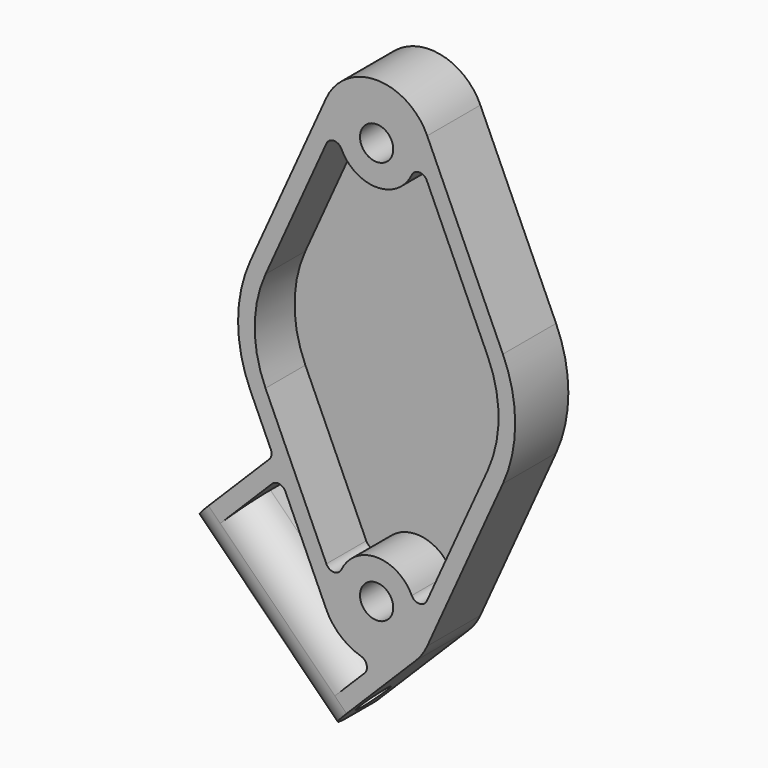
from build123d import *

# Parameters (mm, degrees)
F0_R     = 2
F1_DEPTH = 8
F2_DEPTH = 2
F3_R     = 1
F5_D     = 4
F6_R     = 3.99999


# Not quite as in the source:
# - a fillet or chamfer is up to 0.001 mm smaller than in the source, because OpenCascade refuses the exact size


with BuildPart() as f1:
    # F0 (on Front) → F1 (new body)
    with BuildSketch(Plane.XZ):
        with BuildLine():
            Line((15.1970139668, 6.8636525628), (6.0880650012, 27.0320429916))
            ThreePointArc((6.0880650012, 27.0320429916), (0, 30.9626), (-6.0880650012, 27.0320429916))
            Line((-6.0880650012, 27.0320429916), (-15.1970139668, 6.8636525628))
            ThreePointArc((-15.1970139668, 6.8636525628), (-16.6751, 0), (-15.1970139668, -6.8636525628))
            Line((-15.1970139668, -6.8636525628), (-12.4500889322, -12.9456996558))
            Line((-12.4500889322, -12.9456996558), (-11.570090993, -14.8941288413))
            Line((-11.570090993, -14.8941288413), (-6.0880650012, -27.0320429916))
            ThreePointArc((-6.0880650012, -27.0320429916), (-3.6489564687, -29.8779507977), (-0.0611180905, -30.9623204051))
            ThreePointArc((-0.0611180905, -30.9623204051), (2.5281419438, -30.4657300374), (4.7236147197, -29.0060147197))
            ThreePointArc((4.7236147197, -29.0060147197), (5.4952020611, -28.0807978659), (6.0880650012, -27.0320429916))
            Line((6.0880650012, -27.0320429916), (15.1970139668, -6.8636525628))
            ThreePointArc((15.1970139668, -6.8636525628), (16.6751, 0), (15.1970139668, 6.8636525628))
        make_face()
        with Locations((0, -24.2824)):
            Circle(F0_R, mode=Mode.SUBTRACT)
        with BuildLine():
            Line((-13.3742945868, 6.0404308054), (-6.0462846285, 22.2655920687))
            ThreePointArc((-6.0462846285, 22.2655920687), (-5.1436901116, 22.8539427752), (-4.2309206889, 22.2815046593))
            ThreePointArc((-4.2309206889, 22.2815046593), (0, 19.6022), (4.2309206889, 22.2815046593))
            ThreePointArc((4.2309206889, 22.2815046593), (5.1436901116, 22.8539427752), (6.0462846285, 22.2655920687))
            Line((6.0462846285, 22.2655920687), (13.3742945868, 6.0404308054))
            ThreePointArc((13.3742945868, 6.0404308054), (14.6751, 0), (13.3742945868, -6.0404308054))
            Line((13.3742945868, -6.0404308054), (6.0462846285, -22.2655920687))
            ThreePointArc((6.0462846285, -22.2655920687), (5.1436901116, -22.8539427752), (4.2309206889, -22.2815046593))
            ThreePointArc((4.2309206889, -22.2815046593), (0, -19.6022), (-4.2309206889, -22.2815046593))
            ThreePointArc((-4.2309206889, -22.2815046593), (-5.1436901116, -22.8539427752), (-6.0462846285, -22.2655920687))
            Line((-6.0462846285, -22.2655920687), (-13.3742945868, -6.0404308054))
            ThreePointArc((-13.3742945868, -6.0404308054), (-14.6751, 0), (-13.3742945868, 6.0404308054))
        make_face(mode=Mode.SUBTRACT)
        with Locations((0, 24.2824)):
            Circle(F0_R, mode=Mode.SUBTRACT)
        with BuildLine():
            Line((-11.570090993, -14.8941288413), (-12.4500889322, -12.9456996558))
            Line((-12.4500889322, -12.9456996558), (-23.05669065, -23.5523013736))
            Line((-23.05669065, -23.5523013736), (-6.4396812921, -40.1693107315))
            Line((-6.4396812921, -40.1693107315), (4.7236147197, -29.0060147197))
            ThreePointArc((4.7236147197, -29.0060147197), (2.5281419438, -30.4657300374), (-0.0611180905, -30.9623204051))
            Line((-0.0611180905, -30.9623204051), (-2.197040605, -33.0982429196))
            Line((-2.197040605, -33.0982429196), (-15.9856228381, -19.3096606865))
            Line((-15.9856228381, -19.3096606865), (-11.570090993, -14.8941288413))
        make_face()
    extrude(amount=F1_DEPTH)

    # F0 (on Front) → F2 (join)
    with BuildSketch(Plane.XZ):
        with BuildLine():
            ThreePointArc((-4.2309206889, 22.2815046593), (-5.1436901116, 22.8539427752), (-6.0462846285, 22.2655920687))
            Line((-6.0462846285, 22.2655920687), (-13.3742945868, 6.0404308054))
            ThreePointArc((-13.3742945868, 6.0404308054), (-14.6751, 0), (-13.3742945868, -6.0404308054))
            Line((-13.3742945868, -6.0404308054), (-6.0462846285, -22.2655920687))
            ThreePointArc((-6.0462846285, -22.2655920687), (-5.1436901116, -22.8539427752), (-4.2309206889, -22.2815046593))
            ThreePointArc((-4.2309206889, -22.2815046593), (0, -19.6022), (4.2309206889, -22.2815046593))
            ThreePointArc((4.2309206889, -22.2815046593), (5.1436901116, -22.8539427752), (6.0462846285, -22.2655920687))
            Line((6.0462846285, -22.2655920687), (13.3742945868, -6.0404308054))
            ThreePointArc((13.3742945868, -6.0404308054), (14.6751, 0), (13.3742945868, 6.0404308054))
            Line((13.3742945868, 6.0404308054), (6.0462846285, 22.2655920687))
            ThreePointArc((6.0462846285, 22.2655920687), (5.1436901116, 22.8539427752), (4.2309206889, 22.2815046593))
            ThreePointArc((4.2309206889, 22.2815046593), (0, 19.6022), (-4.2309206889, 22.2815046593))
        make_face()
        with BuildLine():
            Line((-6.0880650012, -27.0320429916), (-11.570090993, -14.8941288413))
            Line((-11.570090993, -14.8941288413), (-15.9856228381, -19.3096606865))
            Line((-15.9856228381, -19.3096606865), (-2.197040605, -33.0982429196))
            Line((-2.197040605, -33.0982429196), (-0.0611180905, -30.9623204051))
            ThreePointArc((-0.0611180905, -30.9623204051), (-3.6489564687, -29.8779507977), (-6.0880650012, -27.0320429916))
        make_face()
    extrude(amount=F2_DEPTH)

    # F3
    f3_edges = [f1.edges().sort_by_distance(p)[0] for p in [
        (-12.450089, -4, -12.9457),
        (-11.570091, -5, -14.894129),
        (-0.061118, -5, -30.96232),
    ]]
    fillet(f3_edges, radius=F3_R)

    # F5 (through all)
    with Locations(Plane(origin=(16.8648147197, 0, -16.8648147197), x_dir=(0, 1, 0), z_dir=(0.7071067812, 0, -0.7071067812))):
        with Locations((-4, -28.9575343242)):
            Hole(F5_D / 2)

    # F6 (radius 4 in the source; OpenCascade refuses exactly that, so slightly less here)
    f6_edges = [f1.edges().sort_by_distance(p)[0] for p in [
        (-14.748186, -8, -31.860806),
        (-9.091332, -8, -26.203952),
    ]]
    fillet(f6_edges, radius=F6_R)


solid = f1.part
